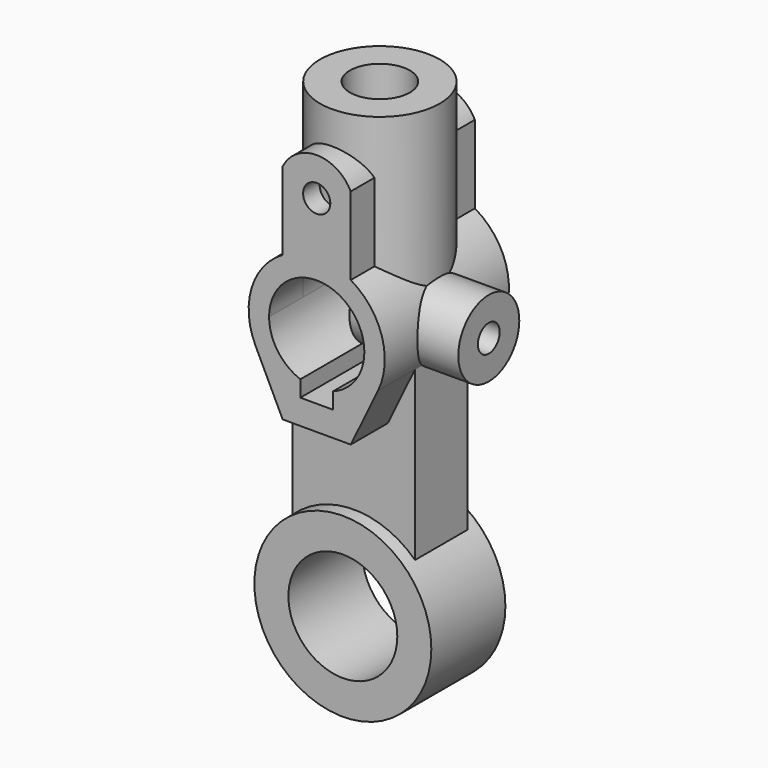
from build123d import *

# Parameters (mm, degrees)
F0_R          = 32.5
F0_R_2        = 20
F1_DEPTH      = 17
F3_DEPTH      = 12
F4_R          = 5
F5_DEPTH      = 40
F5_DEPTH_BACK = 17
F7_DEPTH      = 40.001
F9_R          = 22
F9_R_2        = 11
F10_DEPTH     = 70
F12_DEPTH     = 57.0010001
F13_R         = 14
F13_R_2       = 5
F14_DEPTH     = 40


# Not quite as in the source:
# - a feature names something its author has since deleted; it is built from what else it names


with BuildPart() as f1:
    # F0 (on Front) → F1 (new body, symmetric)
    with BuildSketch(Plane.XZ):
        Circle(F0_R)
        Circle(F0_R_2, mode=Mode.SUBTRACT)
    extrude(amount=F1_DEPTH, both=True)

    # F2 (on Front) → F3 (join, symmetric)
    with BuildSketch(Plane.XZ):
        with BuildLine():
            Line((-22.5, 96), (-22.5, 23.4520787991))
            ThreePointArc((-22.5, 23.4520787991), (0, 32.5), (22.5, 23.4520787991))
            Line((22.5, 23.4520787991), (22.5, 96))
            Line((22.5, 96), (-22.5, 96))
        make_face()
    extrude(amount=F3_DEPTH, both=True)

    # F4 (on face) → F5 (join, two sides)
    with BuildSketch(Plane.XZ.offset(12)) as f5_sk:
        with BuildLine():
            Line((22.5, 96), (22.5, 85.1027526411))
            ThreePointArc((22.5, 85.1027526411), (23.897513742, 103.3422637483), (12.5, 117.6506350946))
            Line((12.5, 117.6506350946), (12.5, 146.3047601065))
            ThreePointArc((12.5, 146.3047601065), (0, 154), (-12.5, 146.3047601065))
            Line((-12.5, 146.3047601065), (-12.5, 117.6506350946))
            ThreePointArc((-12.5, 117.6506350946), (-23.897513742, 103.3422637483), (-22.5, 85.1027526411))
            Line((-22.5, 85.1027526411), (-22.5, 96))
            Line((-22.5, 96), (-17.5, 96))
            ThreePointArc((-17.5, 96), (0, 113.5), (17.5, 96))
            Line((17.5, 96), (22.5, 96))
        make_face()
        with Locations((0, 140)):
            Circle(F4_R, mode=Mode.SUBTRACT)
        with BuildLine():
            Line((-12.5, 64.4553365928), (12.5, 64.4553365928))
            Line((12.5, 64.4553365928), (22.5, 85.1027526411))
            Line((22.5, 85.1027526411), (22.5, 96))
            Line((22.5, 96), (17.5, 96))
            ThreePointArc((17.5, 96), (14.3396303997, 85.9687986761), (6, 79.5607177772))
            Line((6, 79.5607177772), (6, 73.6))
            Line((6, 73.6), (-6, 73.6))
            Line((-6, 73.6), (-6, 79.5607177772))
            ThreePointArc((-6, 79.5607177772), (-14.3396303997, 85.9687986761), (-17.5, 96))
            Line((-17.5, 96), (-22.5, 96))
            Line((-22.5, 96), (-22.5, 85.1027526411))
            Line((-22.5, 85.1027526411), (-12.5, 64.4553365928))
        make_face()
    extrude(amount=-F5_DEPTH)
    extrude(f5_sk.sketch, amount=F5_DEPTH_BACK)

    # F6: union 

    # F7 (cut, through all): a face of the model
    f7_faces = [f1.faces().sort_by_distance(p)[0] for p in [
        (0, -12, 87.144181228),
    ]]
    extrude(f7_faces, amount=-F7_DEPTH, mode=Mode.SUBTRACT)

    # F9 (on face) → F10 (join)
    with BuildSketch(Plane(origin=(0, 0, 96), x_dir=(1, 0, 0), z_dir=(0, 0, -1))):
        Circle(F9_R)
        Circle(F9_R_2, mode=Mode.SUBTRACT)
    extrude(amount=-F10_DEPTH)

    # F11 (on face) → F12 (cut, through all)
    with BuildSketch(Plane.XZ.offset(29)):
        with BuildLine():
            ThreePointArc((17.5, 96), (0, 113.5), (-17.5, 96))
            Line((-17.5, 96), (17.5, 96))
        make_face()
    extrude(amount=-F12_DEPTH, mode=Mode.SUBTRACT)

    # F13 (on Right) → F14 (join)
    with BuildSketch(Plane.YZ):
        with Locations((0, 96)):
            Circle(F13_R)
        with Locations((0, 96)):
            Circle(F13_R_2, mode=Mode.SUBTRACT)
    extrude(amount=F14_DEPTH)


solid = f1.part
